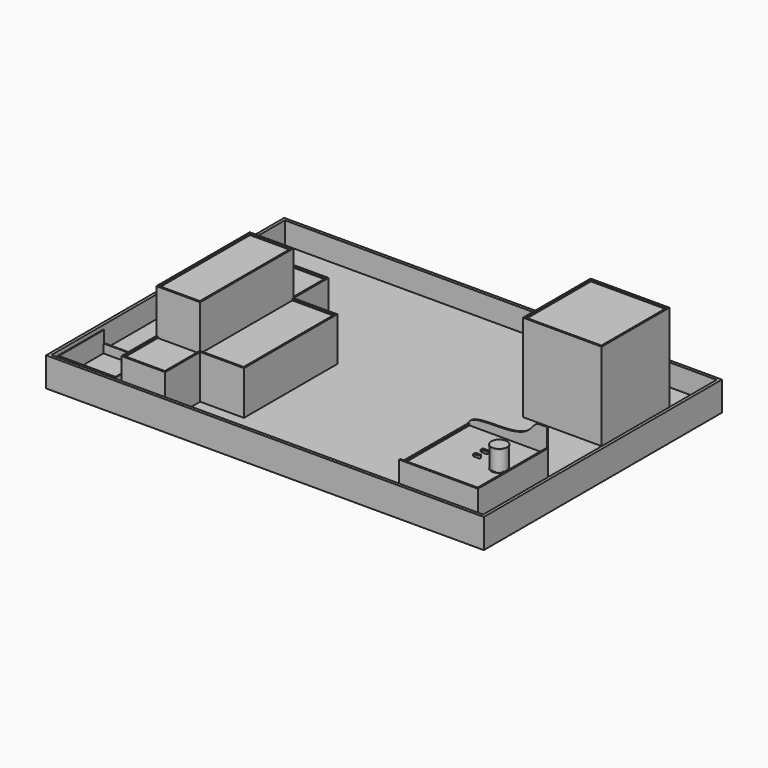
from build123d import *

# Parameters (mm, degrees)
F0_R      = 27.2
F1_DEPTH  = 2.83
F2_R      = 26.4
F3_DEPTH  = 67.36
F4_R      = 27.2
F5_DEPTH  = 2.83
F9_W      = 270
F9_H      = 300
F10_DEPTH = 72
F12_DEPTH = 15
F14_DEPTH = 5
F15_W     = 5
F15_H     = 290
F16_DEPTH = 5
F17_W     = 1500
F17_H     = 1020
F18_DEPTH = 25
F19_W     = 270
F19_H     = 290
F20_DEPTH = 300
F21_W     = 260
F21_H     = 280
F22_DEPTH = 5
F23_W     = 1500
F23_H     = 1020
F23_W_2   = 1480
F23_H_2   = 1000
F24_DEPTH = 75
F26_DEPTH = 150
F27_W     = 150
F27_H     = 400
F28_DEPTH = 150
F29_W     = 140
F29_H     = 390
F30_DEPTH = 5
F31_W     = 140
F31_H     = 145
F31_W_2   = 145
F31_H_2   = 390
F32_DEPTH = 5
F33_R     = 3
F34_DEPTH = 4
F35_R     = 3.99999
F35_2_R   = 3.99999
F36_R     = 3
F37_DEPTH = 8
F38_R     = 3
F39_DEPTH = 8
F40_R     = 3
F40_R_2   = 2.5
F41_DEPTH = 3
F42_R     = 3
F42_R_2   = 2.5
F43_DEPTH = 3
F45_DEPTH = 270.001
F46_W     = 200
F46_H     = 200
F46_W_2   = 194
F46_H_2   = 191
F47_DEPTH = 30
F49_DEPTH = 40


# Not quite as in the source:
# - a fillet or chamfer is up to 0.001 mm smaller than in the source, because OpenCascade refuses the exact size
# - a feature names something its author has since deleted; it is built from what else it names


with BuildPart() as f1:
    # F0 (on Top) → F1 (new body)
    with BuildSketch(Plane.XY):
        Circle(F0_R)
    extrude(amount=F1_DEPTH)

    # F2 (on face) → F3 (join)
    with BuildSketch(Plane.XY.offset(2.83)):
        Circle(F2_R)
    extrude(amount=F3_DEPTH)

    # F4 (on face) → F5 (join)
    with BuildSketch(Plane.XY.offset(70.19)):
        Circle(F4_R)
    extrude(amount=F5_DEPTH)


with BuildPart() as f10:
    # F9 (on Top) → F10 (new body)
    with BuildSketch(Plane.XY):
        with Locations((-87.8, 0)):
            Rectangle(F9_W, F9_H)
    extrude(amount=-F10_DEPTH)

    # F11 (on face) → F12 (join)
    with BuildSketch(Plane.XY):
        Polygon((-222.8, -145), (-222.8, -150), (47.2, -150), (47.2, 150), (42.2, 150), (42.2, -145), align=None)
    extrude(amount=F12_DEPTH)

    # F13 (on face) → F14 (join)
    with BuildSketch(Plane(origin=(0, 150, 0), x_dir=(-1, 0, 0), z_dir=(0, 1, 0))):
        with BuildLine():
            Line((-21.3134280931, 81.3575685024), (-47.2, 81.3575685024))
            Line((-47.2, 81.3575685024), (-47.2, -72))
            Line((-47.2, -72), (222.8, -72))
            Line((222.8, -72), (222.8, 0))
            add(Edge.make_bspline(
                [(-21.3134280931, 81.3575685024), (-6.3059147253, 81.3822787863), (12.9585432644, 38.1268753575), (103.6097013063, 23.6068887567), (223.0224295336, 30.7718731823), (222.8, 0)],
                knots=[0, 0, 0, 0, 0.2487100673, 0.6151112321, 1, 1, 1, 1], degree=3))
        make_face()
    extrude(amount=-F14_DEPTH)

    # F15 (on face) → F16 (join)
    with BuildSketch(Plane.XY):
        with Locations((-220.3, 0)):
            Rectangle(F15_W, F15_H)
    extrude(amount=F16_DEPTH)

    # F17 (on face) → F18 (join)
    with BuildSketch(Plane(origin=(0, 0, -72), x_dir=(1, 0, 0), z_dir=(0, 0, -1))):
        with Locations((-602.8, -260)):
            Rectangle(F17_W, F17_H)
    extrude(amount=F18_DEPTH)

    # F19 (on face) → F20 (join)
    with BuildSketch(Plane.XY.offset(-72)):
        with Locations((-87.8, 525)):
            Rectangle(F19_W, F19_H)
    extrude(amount=F20_DEPTH)

    # F21 (on face) → F22 (cut)
    with BuildSketch(Plane.XY.offset(228)):
        with Locations((-87.8, 525)):
            Rectangle(F21_W, F21_H)
    extrude(amount=-F22_DEPTH, mode=Mode.SUBTRACT)

    # F23 (on face) → F24 (join)
    with BuildSketch(Plane.XY.offset(-72)):
        with Locations((-602.8, 260)):
            Rectangle(F23_W, F23_H)
        with Locations((-602.8, 260)):
            Rectangle(F23_W_2, F23_H_2, mode=Mode.SUBTRACT)
    extrude(amount=F24_DEPTH)

    # F25 (on face) → F26 (join)
    with BuildSketch(Plane.XY.offset(-72)):
        Polygon((-952.8, 460), (-1102.8, 460), (-1102.8, -240), (-952.8, -240), (-952.8, -90), (-802.8, -90), (-802.8, 310), (-952.8, 310), align=None)
    extrude(amount=F26_DEPTH)

    # F27 (on face) → F28 (join)
    with BuildSketch(Plane.XY.offset(78)):
        with Locations((-1027.8, 110)):
            Rectangle(F27_W, F27_H)
    extrude(amount=F28_DEPTH)

    # F29 (on face) → F30 (cut)
    with BuildSketch(Plane.XY.offset(228)):
        with Locations((-1027.8, 110)):
            Rectangle(F29_W, F29_H)
    extrude(amount=-F30_DEPTH, mode=Mode.SUBTRACT)

    # F31 (on face) → F32 (cut)
    with BuildSketch(Plane.XY.offset(78)):
        with Locations((-1027.8, 382.5)):
            Rectangle(F31_W, F31_H)
        with Locations((-880.3, 110)):
            Rectangle(F31_W_2, F31_H_2)
        with Locations((-1027.8, -162.5)):
            Rectangle(F31_W, F31_H)
    extrude(amount=-F32_DEPTH, mode=Mode.SUBTRACT)

    # F46 (on face) → F47 (join)
    with BuildSketch(Plane.XY.offset(-72)):
        with Locations((-1232.8, -130)):
            Rectangle(F46_W, F46_H)
        with Locations((-1232.8, -128.5)):
            Rectangle(F46_W_2, F46_H_2, mode=Mode.SUBTRACT)
    extrude(amount=F47_DEPTH)

    # F48 (on face) → F49 (join)
    with BuildSketch(Plane.XY.offset(-42)):
        Polygon((-1329.8, -30), (-1332.8, -30), (-1332.8, -230), (-1329.8, -230), (-1135.8, -230), (-1132.8, -230), (-1132.8, -30), (-1135.8, -30), (-1135.8, -224), (-1329.8, -224), align=None)
    extrude(amount=F49_DEPTH)


with BuildPart() as f34:
    # F33 (on offset) → F34 (new body, symmetric)
    with BuildSketch(Plane.XY.offset(25)):
        with BuildLine():
            Line((-55, -12), (-74.5, -12))
            Line((-74.5, -12), (-74.5, -13))
            Line((-74.5, -13), (-65.6457513111, -13))
            ThreePointArc((-65.6457513111, -13), (-67, -16), (-65.6457513111, -19))
            Line((-65.6457513111, -19), (-74.5, -19))
            Line((-74.5, -19), (-74.5, -20))
            Line((-74.5, -20), (-55, -20))
            ThreePointArc((-55, -20), (-51, -16), (-55, -12))
        make_face()
        with Locations((-63, -16)):
            Circle(F33_R, mode=Mode.SUBTRACT)
        with Locations((-55, -16)):
            Circle(F33_R, mode=Mode.SUBTRACT)
    extrude(amount=F34_DEPTH, both=True)

    # F35 (radius 4 in the source; OpenCascade refuses exactly that, so slightly less here)
    f35_edges = [f34.edges().sort_by_distance(p)[0] for p in [
        (-74.5, -19.5, 29),
        (-74.5, -12.5, 29),
        (-74.5, -19.5, 21),
        (-74.5, -12.5, 21),
    ]]
    fillet(f35_edges, radius=F35_R)

    # F36 (on face) → F37 (join, through all)
    with BuildSketch(Plane.XZ.offset(20)):
        with Locations((-70.5, 25)):
            Circle(F36_R)
    extrude(amount=-F37_DEPTH)

    # F42 (on offset) → F43 (join, symmetric)
    with BuildSketch(Plane.XY.offset(25)):
        with Locations((-63, -16)):
            Circle(F42_R)
        with Locations((-63, -16)):
            Circle(F42_R_2, mode=Mode.SUBTRACT)
        with Locations((-55, -16)):
            Circle(F42_R)
        with Locations((-55, -16)):
            Circle(F42_R_2, mode=Mode.SUBTRACT)
    extrude(amount=F43_DEPTH, both=True)


with BuildPart() as f34b:
    # F33 (on offset) → F34, piece 2 (new body, symmetric)
    with BuildSketch(Plane.XY.offset(25)):
        with BuildLine():
            Line((-74.5, 13), (-74.5, 12))
            Line((-74.5, 12), (-55, 12))
            ThreePointArc((-55, 12), (-51, 16), (-55, 20))
            Line((-55, 20), (-74.5, 20))
            Line((-74.5, 20), (-74.5, 19))
            Line((-74.5, 19), (-65.6457513111, 19))
            ThreePointArc((-65.6457513111, 19), (-67, 16), (-65.6457513111, 13))
            Line((-65.6457513111, 13), (-74.5, 13))
        make_face()
        with Locations((-63, 16)):
            Circle(F33_R, mode=Mode.SUBTRACT)
        with Locations((-55, 16)):
            Circle(F33_R, mode=Mode.SUBTRACT)
    extrude(amount=F34_DEPTH, both=True)

    # F35#2 (radius 4 in the source; OpenCascade refuses exactly that, so slightly less here)
    f35_2_edges = [f34b.edges().sort_by_distance(p)[0] for p in [
        (-74.5, 12.5, 29),
        (-74.5, 19.5, 29),
        (-74.5, 19.5, 21),
        (-74.5, 12.5, 21),
    ]]
    fillet(f35_2_edges, radius=F35_2_R)

    # F38 (on face) → F39 (join, through all)
    with BuildSketch(Plane(origin=(0, 20, 0), x_dir=(-1, 0, 0), z_dir=(0, 1, 0))):
        with Locations((70.5, 25)):
            Circle(F38_R)
    extrude(amount=-F39_DEPTH)

    # F40 (on offset) → F41 (join, symmetric)
    with BuildSketch(Plane.XY.offset(25)):
        with Locations((-55, 16)):
            Circle(F40_R)
        with Locations((-55, 16)):
            Circle(F40_R_2, mode=Mode.SUBTRACT)
        with Locations((-63, 16)):
            Circle(F40_R)
        with Locations((-63, 16)):
            Circle(F40_R_2, mode=Mode.SUBTRACT)
    extrude(amount=F41_DEPTH, both=True)


with BuildPart() as f45_tool:
    # F44 (on face) → F45 (new body, through all)
    with BuildSketch(Plane(origin=(0, 20, 0), x_dir=(-1, 0, 0), z_dir=(0, 1, 0))):
        with BuildLine():
            Line((71.5, 26), (71.5, 27.2912878475))
            ThreePointArc((71.5, 27.2912878475), (70.5, 27.5), (69.5, 27.2912878475))
            Line((69.5, 27.2912878475), (69.5, 26))
            Line((69.5, 26), (68.2087121525, 26))
            ThreePointArc((68.2087121525, 26), (68, 25), (68.2087121525, 24))
            Line((68.2087121525, 24), (69.5, 24))
            Line((69.5, 24), (69.5, 22.7087121525))
            ThreePointArc((69.5, 22.7087121525), (70.5, 22.5), (71.5, 22.7087121525))
            Line((71.5, 22.7087121525), (71.5, 24))
            Line((71.5, 24), (72.7912878475, 24))
            ThreePointArc((72.7912878475, 24), (73, 25), (72.7912878475, 26))
            Line((72.7912878475, 26), (71.5, 26))
        make_face()
    extrude(amount=-F45_DEPTH)


with BuildPart() as f34_1:
    add(f34.part)

    # F45: cut by f45_tool
    add(f45_tool.part, mode=Mode.SUBTRACT)


with BuildPart() as f34b_1:
    add(f34b.part)

    # F45: cut by f45_tool
    add(f45_tool.part, mode=Mode.SUBTRACT)


solid = Compound([f1.part, f10.part, f34_1.part, f34b_1.part])
